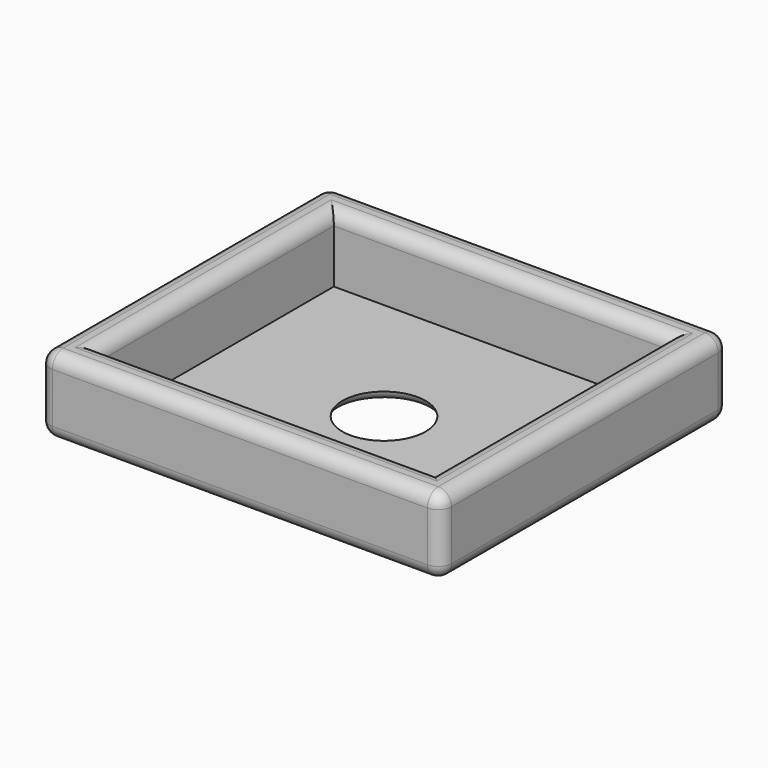
from build123d import *

# Parameters (mm, degrees)
F0_W          = 30.607
F0_H          = 27.432
F0_W_2        = 25.527
F0_H_2        = 22.352
F1_DEPTH      = 5.08
F2_W          = 30.607
F2_H          = 27.432
F2_R          = 3.175
F3_DEPTH      = 0.762
F4_T1_DEPTH   = 3.81
F4_T3_DEPTH   = 28.575
F4_T5_DEPTH   = 25.4
F4_T7_DEPTH   = 22.352
F4_T9_DEPTH   = 25.527
F4_S13_W      = 1.03632
F4_S13_H      = 1.03632
F4_T14_DEPTH  = 1.03632
F4_S19_W      = 1.03632
F4_S19_H      = 1.03632
F4_T20_DEPTH  = 1.03632
F4_S25_W      = 1.03632
F4_S25_H      = 1.03632
F4_T26_DEPTH  = 1.03632
F4_S31_W      = 1.03632
F4_S31_H      = 1.03632
F4_T32_DEPTH  = 1.03632
F4_S37_W      = 1.03632
F4_S37_H      = 1.03632
F4_T38_DEPTH  = 1.03632
F4_S43_W      = 1.03632
F4_S43_H      = 1.03632
F4_T44_DEPTH  = 1.03632
F4_S49_W      = 1.03632
F4_S49_H      = 1.03632
F4_T50_DEPTH  = 1.03632
F4_S55_W      = 1.03632
F4_S55_H      = 1.03632
F4_T56_DEPTH  = 1.03632
F4_T65_DEPTH  = 28.067
F4_T69_DEPTH  = 24.892
F4_T76_DEPTH  = 24.892
F4_T80_DEPTH  = 28.067
F4_T87_DEPTH  = 24.892
F4_T91_DEPTH  = 28.067
F4_T98_DEPTH  = 24.892
F4_T102_DEPTH = 28.067


# Not quite as in the source:
# - a fillet or chamfer that OpenCascade refuses, or shapes differently, is made with other operations: its cross-section is extruded or revolved along the edge and cut away or added


with BuildPart() as f1:
    # F0 (on Top) → F1 (new body)
    with BuildSketch(Plane.XY):
        Rectangle(F0_W, F0_H)
        Rectangle(F0_W_2, F0_H_2, mode=Mode.SUBTRACT)
    extrude(amount=F1_DEPTH)

    # F2 (on face) → F3 (join)
    with BuildSketch(Plane(origin=(0, 0, 0), x_dir=(1, 0, 0), z_dir=(0, 0, -1))):
        Rectangle(F2_W, F2_H)
        Circle(F2_R, mode=Mode.SUBTRACT)
    extrude(amount=F3_DEPTH)

    # F4: fillet of radius 1.016 on 17 edges, made by hand

    # F4_s2 → F4_t1 (cut)
    with BuildSketch(Plane.XY.offset(0.254)):
        with BuildLine():
            ThreePointArc((-14.2875, -13.716), (-15.0059204897, -13.4184204897), (-15.3035, -12.7))
            Line((-15.3035, -12.7), (-15.3035, -13.716))
            Line((-15.3035, -13.716), (-14.2875, -13.716))
        make_face()
        with BuildLine():
            ThreePointArc((14.2875, -13.716), (15.0059204897, -13.4184204897), (15.3035, -12.7))
            Line((15.3035, -12.7), (15.3035, -13.716))
            Line((15.3035, -13.716), (14.2875, -13.716))
        make_face()
        with BuildLine():
            ThreePointArc((-14.2875, 13.716), (-15.0059204897, 13.4184204897), (-15.3035, 12.7))
            Line((-15.3035, 12.7), (-15.3035, 13.716))
            Line((-15.3035, 13.716), (-14.2875, 13.716))
        make_face()
        with BuildLine():
            ThreePointArc((14.2875, 13.716), (15.0059204897, 13.4184204897), (15.3035, 12.7))
            Line((15.3035, 12.7), (15.3035, 13.716))
            Line((15.3035, 13.716), (14.2875, 13.716))
        make_face()
    extrude(amount=F4_T1_DEPTH, mode=Mode.SUBTRACT)

    # F4_s4 → F4_t3 (cut)
    with BuildSketch(Plane.YZ.offset(-14.2875)):
        with BuildLine():
            ThreePointArc((-13.716, 4.064), (-13.4184204897, 4.7824204897), (-12.7, 5.08))
            Line((-12.7, 5.08), (-13.716, 5.08))
            Line((-13.716, 5.08), (-13.716, 4.064))
        make_face()
        with BuildLine():
            ThreePointArc((-13.716, 0.254), (-13.4184204897, -0.4644204897), (-12.7, -0.762))
            Line((-12.7, -0.762), (-13.716, -0.762))
            Line((-13.716, -0.762), (-13.716, 0.254))
        make_face()
        with BuildLine():
            ThreePointArc((12.7, -0.762), (13.4184204897, -0.4644204897), (13.716, 0.254))
            Line((13.716, 0.254), (13.716, -0.762))
            Line((13.716, -0.762), (12.7, -0.762))
        make_face()
        with BuildLine():
            ThreePointArc((13.716, 4.064), (13.4184204897, 4.7824204897), (12.7, 5.08))
            Line((12.7, 5.08), (13.716, 5.08))
            Line((13.716, 5.08), (13.716, 4.064))
        make_face()
    extrude(amount=F4_T3_DEPTH, mode=Mode.SUBTRACT)

    # F4_s6 → F4_t5 (cut)
    with BuildSketch(Plane.XZ.offset(-12.7)):
        with BuildLine():
            ThreePointArc((-14.2875, -0.762), (-15.0059204897, -0.4644204897), (-15.3035, 0.254))
            Line((-15.3035, 0.254), (-15.3035, -0.762))
            Line((-15.3035, -0.762), (-14.2875, -0.762))
        make_face()
        with BuildLine():
            ThreePointArc((14.2875, -0.762), (15.0059204897, -0.4644204897), (15.3035, 0.254))
            Line((15.3035, 0.254), (15.3035, -0.762))
            Line((15.3035, -0.762), (14.2875, -0.762))
        make_face()
        with BuildLine():
            ThreePointArc((-14.2875, 5.08), (-15.0059204897, 4.7824204897), (-15.3035, 4.064))
            Line((-15.3035, 4.064), (-15.3035, 5.08))
            Line((-15.3035, 5.08), (-14.2875, 5.08))
        make_face()
        with BuildLine():
            ThreePointArc((15.3035, 4.064), (15.0059204897, 4.7824204897), (14.2875, 5.08))
            Line((14.2875, 5.08), (15.3035, 5.08))
            Line((15.3035, 5.08), (15.3035, 4.064))
        make_face()
    extrude(amount=F4_T5_DEPTH, mode=Mode.SUBTRACT)

    # F4_s8 → F4_t7 (cut)
    with BuildSketch(Plane.XZ.offset(-11.176)):
        with BuildLine():
            ThreePointArc((-12.7635, 4.064), (-13.0610795103, 4.7824204897), (-13.7795, 5.08))
            Line((-13.7795, 5.08), (-12.7635, 5.08))
            Line((-12.7635, 5.08), (-12.7635, 4.064))
        make_face()
        with BuildLine():
            ThreePointArc((12.7635, 4.064), (13.0610795103, 4.7824204897), (13.7795, 5.08))
            Line((13.7795, 5.08), (12.7635, 5.08))
            Line((12.7635, 5.08), (12.7635, 4.064))
        make_face()
    extrude(amount=F4_T7_DEPTH, mode=Mode.SUBTRACT)

    # F4_s10 → F4_t9 (cut)
    with BuildSketch(Plane.YZ.offset(-12.7635)):
        with BuildLine():
            ThreePointArc((11.176, 4.064), (11.4735795103, 4.7824204897), (12.192, 5.08))
            Line((12.192, 5.08), (11.176, 5.08))
            Line((11.176, 5.08), (11.176, 4.064))
        make_face()
        with BuildLine():
            ThreePointArc((-11.176, 4.064), (-11.4735795103, 4.7824204897), (-12.192, 5.08))
            Line((-12.192, 5.08), (-11.176, 5.08))
            Line((-11.176, 5.08), (-11.176, 4.064))
        make_face()
    extrude(amount=F4_T9_DEPTH, mode=Mode.SUBTRACT)


with BuildPart() as f4_tool12:
    # F4_s13 → F4_t14 (new body)
    with BuildSketch(Plane.XZ.offset(12.7)):
        with Locations((-14.80566, 4.58216)):
            Rectangle(F4_S13_W, F4_S13_H)
    extrude(amount=F4_T14_DEPTH)

    # F4_s15 → F4_t16 (revolve, cut)
    with BuildSketch(Plane(origin=(-14.2875, -12.7, 4.064), x_dir=(0.7071067812, 0, -0.7071067812), z_dir=(-0.7071067812, 0, -0.7071067812))):
        with BuildLine():
            ThreePointArc((0, -1.016), (1.016, 0), (0, 1.016))
            Line((0, 1.016), (0, -1.016))
        make_face()
    revolve(axis=Axis((-14.2875, -12.7, 4.064), (0, -1, 0)), mode=Mode.SUBTRACT)


with BuildPart() as f1_1:
    add(f1.part)

    # F4_t11: cut F4_tool12
    add(f4_tool12.part, mode=Mode.SUBTRACT)


with BuildPart() as f4_tool18:
    # F4_s19 → F4_t20 (new body)
    with BuildSketch(Plane.XZ.offset(12.7)):
        with Locations((-14.80566, -0.26416)):
            Rectangle(F4_S19_W, F4_S19_H)
    extrude(amount=F4_T20_DEPTH)

    # F4_s21 → F4_t22 (revolve, cut)
    with BuildSketch(Plane(origin=(-14.2875, -12.7, 0.254), x_dir=(0.7071067812, 0, 0.7071067812), z_dir=(0.7071067812, 0, -0.7071067812))):
        with BuildLine():
            ThreePointArc((0, -1.016), (1.016, 0), (0, 1.016))
            Line((0, 1.016), (0, -1.016))
        make_face()
    revolve(axis=Axis((-14.2875, -12.7, 0.254), (0, -1, 0)), mode=Mode.SUBTRACT)


with BuildPart() as f1_2:
    add(f1_1.part)

    # F4_t17: cut F4_tool18
    add(f4_tool18.part, mode=Mode.SUBTRACT)


with BuildPart() as f4_tool24:
    # F4_s25 → F4_t26 (new body)
    with BuildSketch(Plane.XZ.offset(12.7)):
        with Locations((14.80566, 4.58216)):
            Rectangle(F4_S25_W, F4_S25_H)
    extrude(amount=F4_T26_DEPTH)

    # F4_s27 → F4_t28 (revolve, cut)
    with BuildSketch(Plane(origin=(14.2875, -12.7, 4.064), x_dir=(-0.7071067812, 0, -0.7071067812), z_dir=(-0.7071067812, 0, 0.7071067812))):
        with BuildLine():
            ThreePointArc((0, -1.016), (1.016, 0), (0, 1.016))
            Line((0, 1.016), (0, -1.016))
        make_face()
    revolve(axis=Axis((14.2875, -12.7, 4.064), (0, -1, 0)), mode=Mode.SUBTRACT)


with BuildPart() as f1_3:
    add(f1_2.part)

    # F4_t23: cut F4_tool24
    add(f4_tool24.part, mode=Mode.SUBTRACT)


with BuildPart() as f4_tool30:
    # F4_s31 → F4_t32 (new body)
    with BuildSketch(Plane.XZ.offset(12.7)):
        with Locations((14.80566, -0.26416)):
            Rectangle(F4_S31_W, F4_S31_H)
    extrude(amount=F4_T32_DEPTH)

    # F4_s33 → F4_t34 (revolve, cut)
    with BuildSketch(Plane(origin=(14.2875, -12.7, 0.254), x_dir=(-0.7071067812, 0, 0.7071067812), z_dir=(0.7071067812, 0, 0.7071067812))):
        with BuildLine():
            ThreePointArc((0, -1.016), (1.016, 0), (0, 1.016))
            Line((0, 1.016), (0, -1.016))
        make_face()
    revolve(axis=Axis((14.2875, -12.7, 0.254), (0, -1, 0)), mode=Mode.SUBTRACT)


with BuildPart() as f1_4:
    add(f1_3.part)

    # F4_t29: cut F4_tool30
    add(f4_tool30.part, mode=Mode.SUBTRACT)


with BuildPart() as f4_tool36:
    # F4_s37 → F4_t38 (new body)
    with BuildSketch(Plane.XZ.offset(-12.7)):
        with Locations((-14.80566, -0.26416)):
            Rectangle(F4_S37_W, F4_S37_H)
    extrude(amount=-F4_T38_DEPTH)

    # F4_s39 → F4_t40 (revolve, cut)
    with BuildSketch(Plane(origin=(-14.2875, 12.7, 0.254), x_dir=(0.7071067812, 0, 0.7071067812), z_dir=(-0.7071067812, 0, 0.7071067812))):
        with BuildLine():
            ThreePointArc((0, -1.016), (1.016, 0), (0, 1.016))
            Line((0, 1.016), (0, -1.016))
        make_face()
    revolve(axis=Axis((-14.2875, 12.7, 0.254), (0, 1, 0)), mode=Mode.SUBTRACT)


with BuildPart() as f1_5:
    add(f1_4.part)

    # F4_t35: cut F4_tool36
    add(f4_tool36.part, mode=Mode.SUBTRACT)


with BuildPart() as f4_tool42:
    # F4_s43 → F4_t44 (new body)
    with BuildSketch(Plane.XZ.offset(-12.7)):
        with Locations((14.80566, -0.26416)):
            Rectangle(F4_S43_W, F4_S43_H)
    extrude(amount=-F4_T44_DEPTH)

    # F4_s45 → F4_t46 (revolve, cut)
    with BuildSketch(Plane(origin=(14.2875, 12.7, 0.254), x_dir=(-0.7071067812, 0, 0.7071067812), z_dir=(-0.7071067812, 0, -0.7071067812))):
        with BuildLine():
            ThreePointArc((0, -1.016), (1.016, 0), (0, 1.016))
            Line((0, 1.016), (0, -1.016))
        make_face()
    revolve(axis=Axis((14.2875, 12.7, 0.254), (0, 1, 0)), mode=Mode.SUBTRACT)


with BuildPart() as f1_6:
    add(f1_5.part)

    # F4_t41: cut F4_tool42
    add(f4_tool42.part, mode=Mode.SUBTRACT)


with BuildPart() as f4_tool48:
    # F4_s49 → F4_t50 (new body)
    with BuildSketch(Plane.XZ.offset(-12.7)):
        with Locations((14.80566, 4.58216)):
            Rectangle(F4_S49_W, F4_S49_H)
    extrude(amount=-F4_T50_DEPTH)

    # F4_s51 → F4_t52 (revolve, cut)
    with BuildSketch(Plane(origin=(14.2875, 12.7, 4.064), x_dir=(-0.7071067812, 0, -0.7071067812), z_dir=(0.7071067812, 0, -0.7071067812))):
        with BuildLine():
            ThreePointArc((0, -1.016), (1.016, 0), (0, 1.016))
            Line((0, 1.016), (0, -1.016))
        make_face()
    revolve(axis=Axis((14.2875, 12.7, 4.064), (0, 1, 0)), mode=Mode.SUBTRACT)


with BuildPart() as f1_7:
    add(f1_6.part)

    # F4_t47: cut F4_tool48
    add(f4_tool48.part, mode=Mode.SUBTRACT)


with BuildPart() as f4_tool54:
    # F4_s55 → F4_t56 (new body)
    with BuildSketch(Plane.XZ.offset(-12.7)):
        with Locations((-14.80566, 4.58216)):
            Rectangle(F4_S55_W, F4_S55_H)
    extrude(amount=-F4_T56_DEPTH)

    # F4_s57 → F4_t58 (revolve, cut)
    with BuildSketch(Plane(origin=(-14.2875, 12.7, 4.064), x_dir=(0.7071067812, 0, -0.7071067812), z_dir=(0.7071067812, 0, 0.7071067812))):
        with BuildLine():
            ThreePointArc((0, -1.016), (1.016, 0), (0, 1.016))
            Line((0, 1.016), (0, -1.016))
        make_face()
    revolve(axis=Axis((-14.2875, 12.7, 4.064), (0, 1, 0)), mode=Mode.SUBTRACT)


with BuildPart() as f1_8:
    add(f1_7.part)

    # F4_t53: cut F4_tool54
    add(f4_tool54.part, mode=Mode.SUBTRACT)

    # F4_s59 → F4_t60 (revolve, cut)
    with BuildSketch(Plane.XZ):
        with BuildLine():
            ThreePointArc((4.1587377699, -0.762), (3.5365673753, -0.5492185257), (3.175, 0))
            Line((3.175, 0), (3.175, -0.762))
            Line((3.175, -0.762), (4.1587377699, -0.762))
        make_face()
    revolve(axis=Axis((0, 0, -0.762), (0, 0, -1)), mode=Mode.SUBTRACT)


with BuildPart() as f4_tool63:
    # F4_s64 → F4_t65 (new body)
    with BuildSketch(Plane.YZ.offset(12.7635)):
        with BuildLine():
            ThreePointArc((-11.176, 4.064), (-11.4735795103, 4.7824204897), (-12.192, 5.08))
            Line((-12.192, 5.08), (-11.176, 5.08))
            Line((-11.176, 5.08), (-11.176, 4.064))
        make_face()
    extrude(amount=-F4_T65_DEPTH)

    split(bisect_by=Plane.YZ.offset(-12.7635), keep=Keep.BOTTOM)


with BuildPart() as f4_tool67:
    # F4_s68 → F4_t69 (new body)
    with BuildSketch(Plane.XZ.offset(13.716)):
        with BuildLine():
            ThreePointArc((-12.7635, 4.064), (-13.0610795103, 4.7824204897), (-13.7795, 5.08))
            Line((-13.7795, 5.08), (-12.7635, 5.08))
            Line((-12.7635, 5.08), (-12.7635, 4.064))
        make_face()
    extrude(amount=-F4_T69_DEPTH)

    split(bisect_by=Plane.XZ.offset(11.176), keep=Keep.TOP)


with BuildPart() as f4_tool63_1:
    add(f4_tool63.part)

    # F4_t71: intersect F4_tool67
    add(f4_tool67.part, mode=Mode.INTERSECT)


with BuildPart() as f1_9:
    add(f1_8.part)

    # F4_t61: cut F4_tool63
    add(f4_tool63_1.part, mode=Mode.SUBTRACT)


with BuildPart() as f4_tool74:
    # F4_s75 → F4_t76 (new body)
    with BuildSketch(Plane.XZ.offset(11.176)):
        with BuildLine():
            ThreePointArc((-12.7635, 4.064), (-13.0610795103, 4.7824204897), (-13.7795, 5.08))
            Line((-13.7795, 5.08), (-12.7635, 5.08))
            Line((-12.7635, 5.08), (-12.7635, 4.064))
        make_face()
    extrude(amount=-F4_T76_DEPTH)

    split(bisect_by=Plane.XZ.offset(-11.176), keep=Keep.BOTTOM)


with BuildPart() as f4_tool78:
    # F4_s79 → F4_t80 (new body)
    with BuildSketch(Plane.YZ.offset(-15.3035)):
        with BuildLine():
            ThreePointArc((11.176, 4.064), (11.4735795103, 4.7824204897), (12.192, 5.08))
            Line((12.192, 5.08), (11.176, 5.08))
            Line((11.176, 5.08), (11.176, 4.064))
        make_face()
    extrude(amount=F4_T80_DEPTH)

    split(bisect_by=Plane.YZ.offset(-12.7635), keep=Keep.BOTTOM)


with BuildPart() as f4_tool74_1:
    add(f4_tool74.part)

    # F4_t82: intersect F4_tool78
    add(f4_tool78.part, mode=Mode.INTERSECT)


with BuildPart() as f1_10:
    add(f1_9.part)

    # F4_t72: cut F4_tool74
    add(f4_tool74_1.part, mode=Mode.SUBTRACT)


with BuildPart() as f4_tool85:
    # F4_s86 → F4_t87 (new body)
    with BuildSketch(Plane.XZ.offset(-13.716)):
        with BuildLine():
            ThreePointArc((12.7635, 4.064), (13.0610795103, 4.7824204897), (13.7795, 5.08))
            Line((13.7795, 5.08), (12.7635, 5.08))
            Line((12.7635, 5.08), (12.7635, 4.064))
        make_face()
    extrude(amount=F4_T87_DEPTH)

    split(bisect_by=Plane.XZ.offset(-11.176), keep=Keep.BOTTOM)


with BuildPart() as f4_tool89:
    # F4_s90 → F4_t91 (new body)
    with BuildSketch(Plane.YZ.offset(-12.7635)):
        with BuildLine():
            ThreePointArc((11.176, 4.064), (11.4735795103, 4.7824204897), (12.192, 5.08))
            Line((12.192, 5.08), (11.176, 5.08))
            Line((11.176, 5.08), (11.176, 4.064))
        make_face()
    extrude(amount=F4_T91_DEPTH)

    split(bisect_by=Plane.YZ.offset(12.7635), keep=Keep.TOP)


with BuildPart() as f4_tool85_1:
    add(f4_tool85.part)

    # F4_t93: intersect F4_tool89
    add(f4_tool89.part, mode=Mode.INTERSECT)


with BuildPart() as f1_11:
    add(f1_10.part)

    # F4_t83: cut F4_tool85
    add(f4_tool85_1.part, mode=Mode.SUBTRACT)


with BuildPart() as f4_tool96:
    # F4_s97 → F4_t98 (new body)
    with BuildSketch(Plane.XZ.offset(-11.176)):
        with BuildLine():
            ThreePointArc((12.7635, 4.064), (13.0610795103, 4.7824204897), (13.7795, 5.08))
            Line((13.7795, 5.08), (12.7635, 5.08))
            Line((12.7635, 5.08), (12.7635, 4.064))
        make_face()
    extrude(amount=F4_T98_DEPTH)

    split(bisect_by=Plane.XZ.offset(11.176), keep=Keep.TOP)


with BuildPart() as f4_tool100:
    # F4_s101 → F4_t102 (new body)
    with BuildSketch(Plane.YZ.offset(15.3035)):
        with BuildLine():
            ThreePointArc((-11.176, 4.064), (-11.4735795103, 4.7824204897), (-12.192, 5.08))
            Line((-12.192, 5.08), (-11.176, 5.08))
            Line((-11.176, 5.08), (-11.176, 4.064))
        make_face()
    extrude(amount=-F4_T102_DEPTH)

    split(bisect_by=Plane.YZ.offset(12.7635), keep=Keep.TOP)


with BuildPart() as f4_tool96_1:
    add(f4_tool96.part)

    # F4_t104: intersect F4_tool100
    add(f4_tool100.part, mode=Mode.INTERSECT)


with BuildPart() as f1_12:
    add(f1_11.part)

    # F4_t94: cut F4_tool96
    add(f4_tool96_1.part, mode=Mode.SUBTRACT)


solid = f1_12.part
